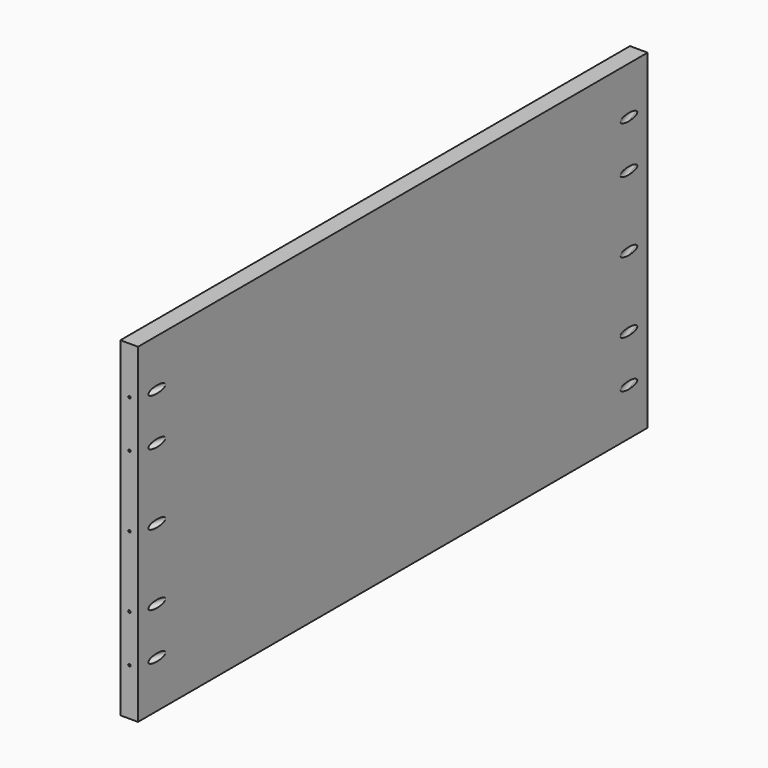
from build123d import *

# Parameters (mm, degrees)
F0_W     = 685.8
F0_H     = 355.6
F1_DEPTH = 19.05
F6_DEPTH = 25.4
F8_D     = 2.54


# Not quite as in the source:
# - a pattern or mirror of a feature is missing from the dataset's text; its kind, count and spacing are read off the source's solid


with BuildPart() as f1:
    # F0 (on Right) → F1 (new body)
    with BuildSketch(Plane.YZ):
        Rectangle(F0_W, F0_H)
    extrude(amount=F1_DEPTH)

    # F5 (on face) → F6 (cut, symmetric)
    with BuildSketch(Plane(origin=(-99.8141063584, -274.2370033629, 0), x_dir=(0.9396926208, -0.3420201433, 0), z_dir=(-0.3420201433, -0.9396926208, 0))):
        with BuildLine():
            ThreePointArc((126.4925399319, -123.063), (122.5555399319, -127), (126.4925399319, -130.937))
            Line((126.4925399319, -130.937), (126.4925399319, -123.063))
        make_face()
        with BuildLine():
            ThreePointArc((126.4925399319, 130.937), (122.5555399319, 127), (126.4925399319, 123.063))
            Line((126.4925399319, 123.063), (126.4925399319, 130.937))
        make_face()
        with BuildLine():
            Line((126.4925399319, 130.937), (126.4925399319, 123.063))
            ThreePointArc((126.4925399319, 123.063), (129.2764193294, 124.2161206025), (130.4295399319, 127))
            ThreePointArc((130.4295399319, 127), (129.2764193294, 129.7838793975), (126.4925399319, 130.937))
        make_face()
        with BuildLine():
            ThreePointArc((126.4925399319, 80.137), (122.5555399319, 76.2), (126.4925399319, 72.263))
            Line((126.4925399319, 72.263), (126.4925399319, 80.137))
        make_face()
        with BuildLine():
            Line((126.4925399319, 80.137), (126.4925399319, 72.263))
            ThreePointArc((126.4925399319, 72.263), (129.2764193294, 73.4161206025), (130.4295399319, 76.2))
            ThreePointArc((130.4295399319, 76.2), (129.2764193294, 78.9838793975), (126.4925399319, 80.137))
        make_face()
        with BuildLine():
            ThreePointArc((126.4925399319, 3.937), (122.5555399319, 0), (126.4925399319, -3.937))
            Line((126.4925399319, -3.937), (126.4925399319, 3.937))
        make_face()
        with BuildLine():
            Line((126.4925399319, 3.937), (126.4925399319, -3.937))
            ThreePointArc((126.4925399319, -3.937), (129.2764193294, -2.7838793975), (130.4295399319, 0))
            ThreePointArc((130.4295399319, 0), (129.2764193294, 2.7838793975), (126.4925399319, 3.937))
        make_face()
        with BuildLine():
            ThreePointArc((126.4925399319, -72.263), (122.5555399319, -76.2), (126.4925399319, -80.137))
            Line((126.4925399319, -80.137), (126.4925399319, -72.263))
        make_face()
        with BuildLine():
            Line((126.4925399319, -72.263), (126.4925399319, -80.137))
            ThreePointArc((126.4925399319, -80.137), (129.2764193294, -78.9838793975), (130.4295399319, -76.2))
            ThreePointArc((130.4295399319, -76.2), (129.2764193294, -73.4161206025), (126.4925399319, -72.263))
        make_face()
        with BuildLine():
            Line((126.4925399319, -123.063), (126.4925399319, -130.937))
            ThreePointArc((126.4925399319, -130.937), (129.2764193294, -129.7838793975), (130.4295399319, -127))
            ThreePointArc((130.4295399319, -127), (129.2764193294, -124.2161206025), (126.4925399319, -123.063))
        make_face()
    f6 = extrude(amount=F6_DEPTH, both=True, mode=Mode.SUBTRACT)

    # F6_copies: F6 across plane
    add(f6.mirror(Plane.ZX.offset(1.1e-05)), mode=Mode.SUBTRACT)

    # F8 (through all)
    with Locations(Plane(origin=(-108.5014179989, -298.1051959308, 0), x_dir=(-0.9396926208, 0.3420201433, 0), z_dir=(0.3420201433, 0.9396926208, 0))):
        with Locations((-126.4925399319, 127), (-126.4925399319, 76.2), (-126.4925399319, 0), (-126.4925399319, -76.2), (-126.4925399319, -127)):
            f8 = Hole(F8_D / 2)

    # F8_copies: F8 across plane
    add(f8.mirror(Plane.ZX.offset(-2e-06)), mode=Mode.SUBTRACT)


solid = f1.part
